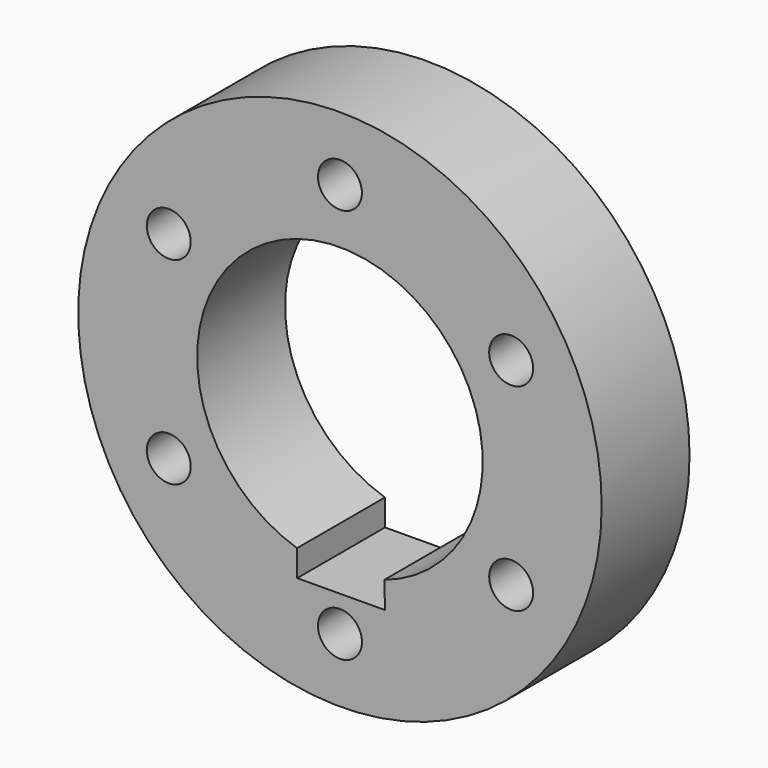
from build123d import *

# Parameters (mm, degrees)
F0_R            = 59.5854737817
F0_R_2          = 5
F1_DEPTH        = 25
F3_D            = 10
F3_DEPTH        = 35
F3_TIP          = 3.0043030951
F3_COPIES_COUNT = 6


# Not quite as in the source:
# - a pattern or mirror of a feature is missing from the dataset's text; its kind, count and spacing are read off the source's solid


with BuildPart() as f1:
    # F0 (on Front) → F1 (new body)
    with BuildSketch(Plane.XZ):
        Circle(F0_R)
        with BuildLine():
            Line((-9.7349431967, -36.997402159), (-9.7675768508, -30.9974909059))
            ThreePointArc((-9.7675768508, -30.9974909059), (-0.1743718668, 32.499532219), (10.099630663, -30.8908960775))
            Line((10.099630663, -30.8908960775), (10.2647609802, -36.8886233119))
            Line((10.2647609802, -36.8886233119), (-9.7349431967, -36.997402159))
        make_face(mode=Mode.SUBTRACT)
        with Locations((0, 45)):
            Circle(F0_R_2, mode=Mode.SUBTRACT)
        with Locations((0, 45)):
            Circle(F0_R_2)
    extrude(amount=F1_DEPTH)

    # F3
    with Locations(Plane.XZ.offset(25)):
        with Locations((0, 45)):
            f3 = Hole(F3_D / 2, depth=F3_DEPTH)
            with Locations((0, 0, -(F3_DEPTH + F3_TIP / 2))):  # 118° drill point
                Cone(0, F3_D / 2, F3_TIP, mode=Mode.SUBTRACT)

    # F3_copies: F3 ×6 about axis
    f3_copies_axis = Axis((0, 0, 0), (0, 1, 0))
    for i in range(1, F3_COPIES_COUNT):
        add(f3.rotate(f3_copies_axis, i * 360 / F3_COPIES_COUNT), mode=Mode.SUBTRACT)


solid = f1.part
